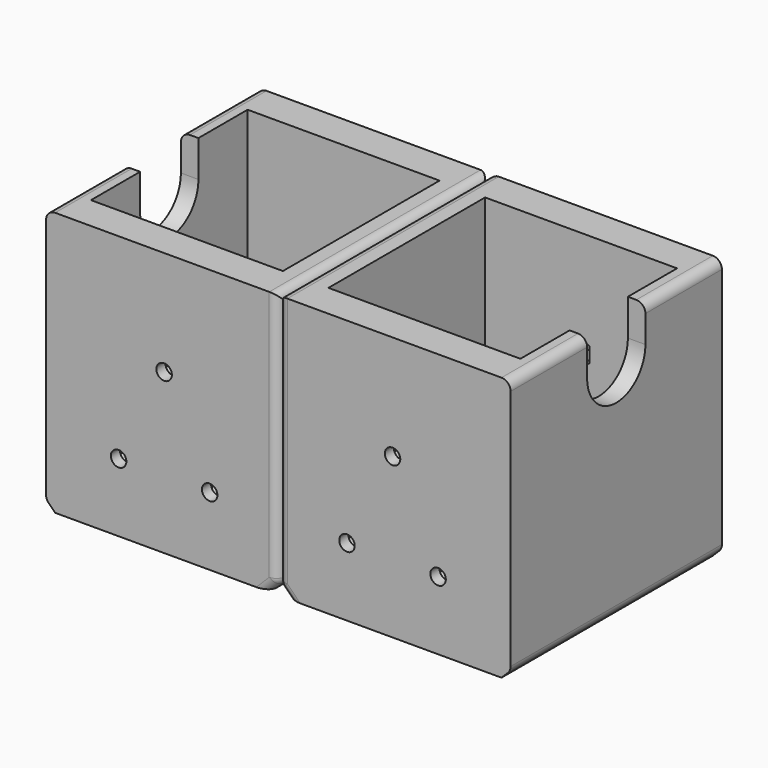
from build123d import *

# Parameters (mm, degrees)
F0_W     = 51
F0_H     = 58
F1_DEPTH = 58
F0_R     = 1.7
F0_R_2   = 11
F0_R_3   = 4.075
F2_DEPTH = 5
F3_R     = 1.7
F4_DEPTH = 99.5
F5_DEPTH = 26.5
F7_DEPTH = 3.85
F8_SIZE  = 2
F9_R     = 2


# Not quite as in the source:
# - two fillets or chamfers of one size are made in one step


with BuildPart() as f1:
    # F0 (on Top) → F1 (new body)
    with BuildSketch(Plane.XY):
        with Locations((0.575, 0)):
            Rectangle(F0_W, F0_H)
        Polygon((-21.075, -21.5), (-21.075, 0), (-21.075, 21.5), (21.075, 21.5), (21.075, 0), (21.075, -21.5), align=None, mode=Mode.SUBTRACT)
    extrude(amount=F1_DEPTH)

    # F0 (on Top) → F2 (join)
    with BuildSketch(Plane.XY):
        with Locations((0.575, 0)):
            Rectangle(F0_W, F0_H)
        Polygon((-21.075, -21.5), (-21.075, 0), (-21.075, 21.5), (21.075, 21.5), (21.075, 0), (21.075, -21.5), align=None, mode=Mode.SUBTRACT)
        Polygon((-21.075, 21.5), (-21.075, 0), (-21.075, -21.5), (21.075, -21.5), (21.075, 0), (21.075, 21.5), align=None)
        with Locations((-15.5, -15.5)):
            Circle(F0_R, mode=Mode.SUBTRACT)
        with Locations((15.5, -15.5)):
            Circle(F0_R, mode=Mode.SUBTRACT)
        with BuildLine():
            ThreePointArc((-21.075, 0), (-17, 4.075), (-12.925, 0))
            ThreePointArc((-12.925, 0), (-17, -4.075), (-21.075, 0))
        make_face(mode=Mode.SUBTRACT)
        Circle(F0_R_2, mode=Mode.SUBTRACT)
        with Locations((-15.5, 15.5)):
            Circle(F0_R, mode=Mode.SUBTRACT)
        with Locations((17, 0)):
            Circle(F0_R_3, mode=Mode.SUBTRACT)
        with Locations((15.5, 15.5)):
            Circle(F0_R, mode=Mode.SUBTRACT)
    extrude(amount=F2_DEPTH)

    # F3 (on Front) → F4 (cut, symmetric)
    with BuildSketch(Plane.XZ):
        with Locations((1, 35)):
            Circle(F3_R)
        with Locations((11, 15)):
            Circle(F3_R)
        with Locations((-9, 15)):
            Circle(F3_R)
    extrude(amount=F4_DEPTH, both=True, mode=Mode.SUBTRACT)

    # F3 (on Front) → F5 (cut, symmetric)
    with BuildSketch(Plane.XZ):
        Polygon((-1.85, 36.6454482672), (-1.85, 33.3545517328), (1, 31.7091034656), (3.85, 33.3545517328), (3.85, 36.6454482672), (1, 38.2908965344), align=None)
        with Locations((1, 35)):
            Circle(F3_R, mode=Mode.SUBTRACT)
        Polygon((11, 18.2908965344), (8.15, 16.6454482672), (8.15, 13.3545517328), (11, 11.7091034656), (13.85, 13.3545517328), (13.85, 16.6454482672), align=None)
        with Locations((11, 15)):
            Circle(F3_R, mode=Mode.SUBTRACT)
        Polygon((-6.15, 13.3545517328), (-6.15, 16.6454482672), (-9, 18.2908965344), (-11.85, 16.6454482672), (-11.85, 13.3545517328), (-9, 11.7091034656), align=None)
        with Locations((-9, 15)):
            Circle(F3_R, mode=Mode.SUBTRACT)
    extrude(amount=F5_DEPTH, both=True, mode=Mode.SUBTRACT)

    # F6 (on face) → F7 (cut, through all)
    with BuildSketch(Plane(origin=(-24.925, 0, 0), x_dir=(0, -1, 0), z_dir=(-1, 0, 0))):
        with BuildLine():
            Line((8, 50), (8, 58))
            Line((8, 58), (-8, 58))
            Line((-8, 58), (-8, 50))
            ThreePointArc((-8, 50), (0, 42), (8, 50))
        make_face()
    extrude(amount=-F7_DEPTH, mode=Mode.SUBTRACT)

    # F8
    f8_edges = [f1.edges().sort_by_distance(p)[0] for p in [
        (-24.925, 0, 0),
        (26.075, 0, 0),
    ]]
    chamfer(f8_edges, length=F8_SIZE)

    # F9
    f9_edges = [f1.edges().sort_by_distance(p)[0] for p in [
        (26.075, 0, 2),
        (-24.925, 0, 2),
        (25.075, 29, 1),
        (26.075, 29, 30),
        (25.075, -29, 1),
        (26.075, -29, 30),
        (26.075, 0, 58),
        (-24.925, -18.5, 58),
        (-24.925, 18.5, 58),
    ]]
    fillet(f9_edges, radius=F9_R)


with BuildPart() as f11_1:
    # F11: instance of F1
    add(f1.part.mirror(Plane(origin=(26.075, 0, 29.4142135624), x_dir=(0, 1, 0), z_dir=(1, 0, 0))))


solid = Compound([f1.part, f11_1.part])
